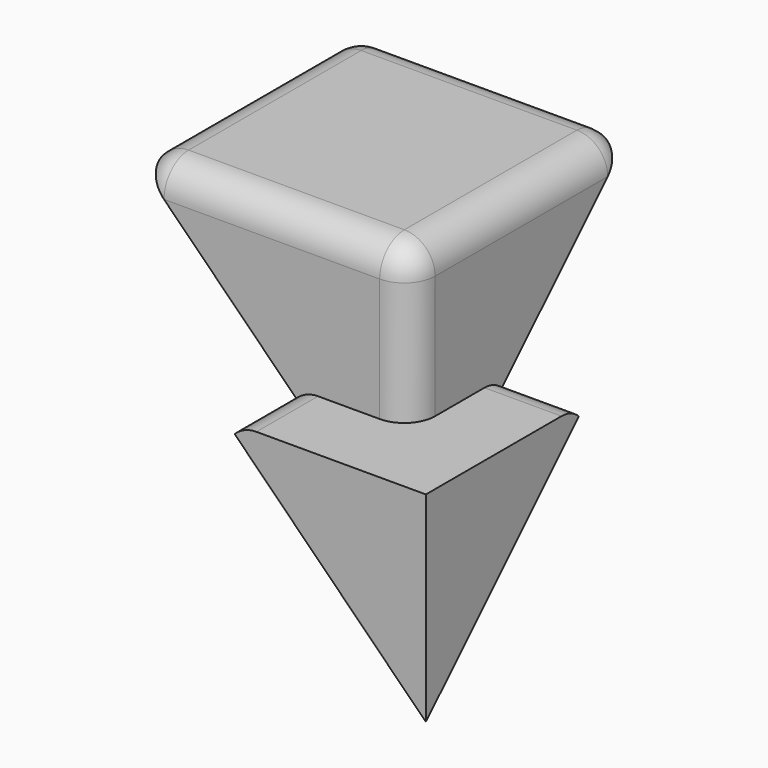
from build123d import *

# Parameters (mm, degrees)
F0_W         = 18
F0_H         = 18
F1_DEPTH     = 18
F2_W         = 10
F2_H         = 10
F2_W_2       = 3
F2_H_2       = 3
F3_DEPTH     = 5
F4_DEPTH     = 8
F5_R         = 2
F6_R         = 2
F7_T1_DEPTH  = 8
F7_T3_DEPTH  = 8
F7_T5_DEPTH  = 8
F7_S9_W      = 2
F7_S9_H      = 2
F7_T10_DEPTH = 2
F7_S15_W     = 2
F7_S15_H     = 2
F7_T16_DEPTH = 2
F7_S21_W     = 2
F7_S21_H     = 2
F7_T22_DEPTH = 2
F8_R         = 2
F10_DEPTH    = 20
F12_DEPTH    = 20


# Not quite as in the source:
# - a fillet or chamfer that OpenCascade refuses, or shapes differently, is made with other operations: its cross-section is extruded or revolved along the edge and cut away or added


with BuildPart() as f1:
    # F0 (on Front) → F1 (new body)
    with BuildSketch(Plane.XZ):
        with Locations((-9, 9)):
            Rectangle(F0_W, F0_H)
    extrude(amount=-F1_DEPTH)

    # F2 (on Top) → F3 (join)
    with BuildSketch(Plane.XY):
        Rectangle(F2_W, F2_H)
        with Locations((-6.5, 0)):
            Rectangle(F2_W_2, F2_H)
        with Locations((0, 6.5)):
            Rectangle(F2_W, F2_H_2)
        with Locations((-6.5, 6.5)):
            Rectangle(F2_W_2, F2_H_2)
    extrude(amount=-F3_DEPTH)

    # F2 (on Top) → F4 (join)
    with BuildSketch(Plane.XY):
        Rectangle(F2_W, F2_H)
        with Locations((-6.5, 0)):
            Rectangle(F2_W_2, F2_H)
        with Locations((0, 6.5)):
            Rectangle(F2_W, F2_H_2)
        with Locations((-6.5, 6.5)):
            Rectangle(F2_W_2, F2_H_2)
    extrude(amount=F4_DEPTH)

    # F5
    f5_edges = [f1.edges().sort_by_distance(p)[0] for p in [
        (-18, 18, 9),
        (-18, 9, 18),
        (-9, 18, 18),
    ]]
    fillet(f5_edges, radius=F5_R)

    # F6
    f6_edges = [f1.edges().sort_by_distance(p)[0] for p in [
        (0, 8, 18),
        (-8, 0, 18),
        (-18, 8, 0),
    ]]
    fillet(f6_edges, radius=F6_R)

    # F7: fillet of radius 2 on 3 edges, made by hand

    # F7_s2 → F7_t1 (cut)
    with BuildSketch(Plane.XZ.offset(-16)):
        with BuildLine():
            ThreePointArc((-2, 0), (-0.5857864376, 0.5857864376), (0, 2))
            Line((0, 2), (0, 0))
            Line((0, 0), (-2, 0))
        make_face()
    extrude(amount=F7_T1_DEPTH, mode=Mode.SUBTRACT)

    # F7_s4 → F7_t3 (cut)
    with BuildSketch(Plane.XY.offset(8)):
        with BuildLine():
            ThreePointArc((0, 2), (-0.5857864376, 0.5857864376), (-2, 0))
            Line((-2, 0), (0, 0))
            Line((0, 0), (0, 2))
        make_face()
    extrude(amount=F7_T3_DEPTH, mode=Mode.SUBTRACT)

    # F7_s6 → F7_t5 (cut)
    with BuildSketch(Plane.YZ.offset(-16)):
        with BuildLine():
            ThreePointArc((2, 0), (0.5857864376, 0.5857864376), (0, 2))
            Line((0, 2), (0, 0))
            Line((0, 0), (2, 0))
        make_face()
    extrude(amount=F7_T5_DEPTH, mode=Mode.SUBTRACT)


with BuildPart() as f7_tool8:
    # F7_s9 → F7_t10 (new body)
    with BuildSketch(Plane.XY.offset(2)):
        with Locations((-17, 1)):
            Rectangle(F7_S9_W, F7_S9_H)
    extrude(amount=-F7_T10_DEPTH)

    # F7_s11 → F7_t12 (revolve, cut)
    with BuildSketch(Plane(origin=(-16, 2, 2), x_dir=(0.7071067812, 0.7071067812, 0), z_dir=(-0.7071067812, 0.7071067812, 0))):
        with BuildLine():
            ThreePointArc((0, -2), (2, 0), (0, 2))
            Line((0, 2), (0, -2))
        make_face()
    revolve(axis=Axis((-16, 2, 2), (0, 0, -1)), mode=Mode.SUBTRACT)


with BuildPart() as f1_1:
    add(f1.part)

    # F7_t7: cut F7_tool8
    add(f7_tool8.part, mode=Mode.SUBTRACT)


with BuildPart() as f7_tool14:
    # F7_s15 → F7_t16 (new body)
    with BuildSketch(Plane.YZ.offset(-2)):
        with Locations((1, 17)):
            Rectangle(F7_S15_W, F7_S15_H)
    extrude(amount=F7_T16_DEPTH)

    # F7_s17 → F7_t18 (revolve, cut)
    with BuildSketch(Plane(origin=(-2, 2, 16), x_dir=(0, 0.7071067812, -0.7071067812), z_dir=(0, -0.7071067812, -0.7071067812))):
        with BuildLine():
            ThreePointArc((0, -2), (2, 0), (0, 2))
            Line((0, 2), (0, -2))
        make_face()
    revolve(axis=Axis((-2, 2, 16), (1, 0, 0)), mode=Mode.SUBTRACT)


with BuildPart() as f1_2:
    add(f1_1.part)

    # F7_t13: cut F7_tool14
    add(f7_tool14.part, mode=Mode.SUBTRACT)


with BuildPart() as f7_tool20:
    # F7_s21 → F7_t22 (new body)
    with BuildSketch(Plane.XY.offset(2)):
        with Locations((-1, 17)):
            Rectangle(F7_S21_W, F7_S21_H)
    extrude(amount=-F7_T22_DEPTH)

    # F7_s23 → F7_t24 (revolve, cut)
    with BuildSketch(Plane(origin=(-2, 16, 2), x_dir=(-0.7071067812, -0.7071067812, 0), z_dir=(0.7071067812, -0.7071067812, 0))):
        with BuildLine():
            ThreePointArc((0, -2), (2, 0), (0, 2))
            Line((0, 2), (0, -2))
        make_face()
    revolve(axis=Axis((-2, 16, 2), (0, 0, -1)), mode=Mode.SUBTRACT)


with BuildPart() as f1_3:
    add(f1_2.part)

    # F7_t19: cut F7_tool20
    add(f7_tool20.part, mode=Mode.SUBTRACT)

    # F8
    f8_edges = [f1_3.edges().sort_by_distance(p)[0] for p in [
        (-8, -2.5, 8),
        (2.5, 8, 8),
        (-8, 8, -2.5),
    ]]
    fillet(f8_edges, radius=F8_R)

    # F9 (on Front) → F10 (cut, symmetric)
    with BuildSketch(Plane.XZ):
        Polygon((5, -5), (-18, 18), (-18, -5), align=None)
    extrude(amount=F10_DEPTH, both=True, mode=Mode.SUBTRACT)

    # F11 (on Right) → F12 (cut, symmetric)
    with BuildSketch(Plane.YZ):
        Polygon((18, 18), (-5, -5), (18, -5), align=None)
    extrude(amount=F12_DEPTH, both=True, mode=Mode.SUBTRACT)


solid = f1_3.part
